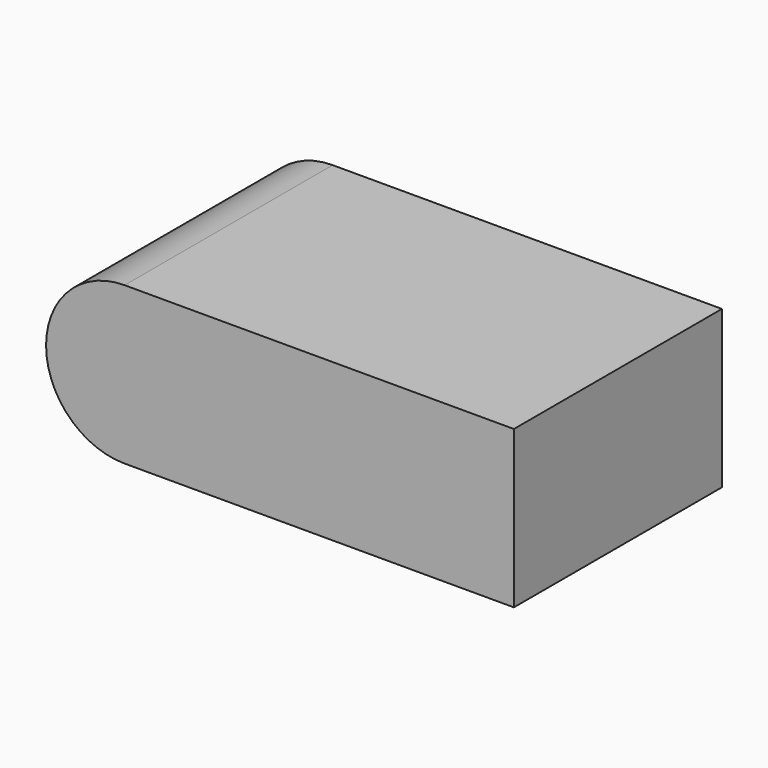
from build123d import *

# Parameters (mm, degrees)
F0_W     = 54.69
F0_H     = 18.36
F1_DEPTH = 30.4
F2_R     = 9.17999


# Not quite as in the source:
# - a fillet or chamfer is up to 0.001 mm smaller than in the source, because OpenCascade refuses the exact size


with BuildPart() as f1:
    # F0 (on Front) → F1 (new body)
    with BuildSketch(Plane.XZ):
        Rectangle(F0_W, F0_H)
    extrude(amount=F1_DEPTH)

    # F2 (radius 9.18 in the source; OpenCascade refuses exactly that, so slightly less here)
    f2_edges = [f1.edges().sort_by_distance(p)[0] for p in [
        (-27.345, -15.2, 9.18),
        (-27.345, -15.2, -9.18),
    ]]
    fillet(f2_edges, radius=F2_R)


solid = f1.part
